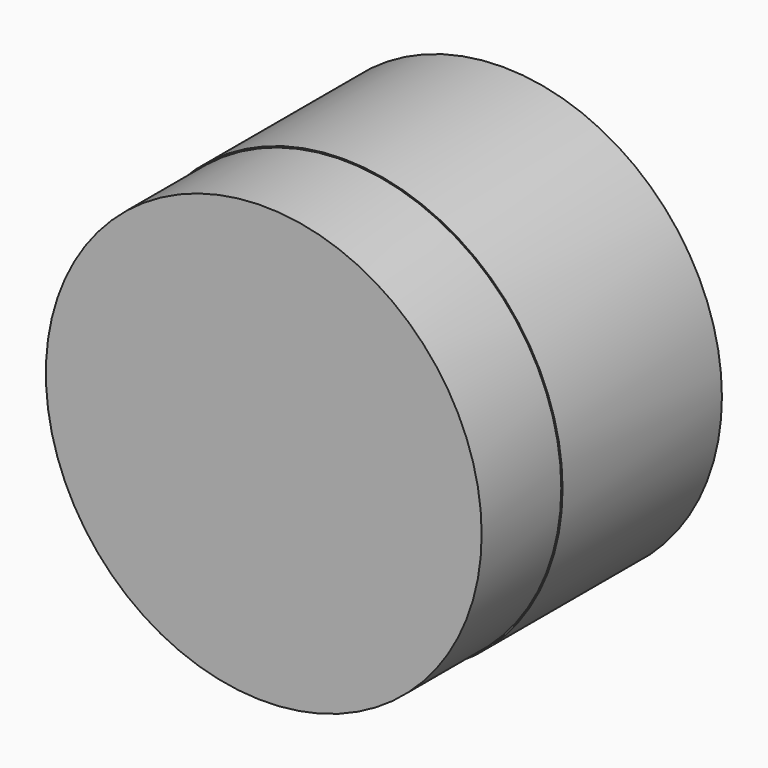
from build123d import *

# Parameters (mm, degrees)
F1_START = 20
F0_R     = 44
F0_R_2   = 30
F1_DEPTH = 40
F3_START = 60.01
F2_R     = 43.7564133354
F3_DEPTH = 19.99


with BuildPart() as f1:
    # F0 (on Front) → F1 (new body)
    with BuildSketch(Plane.XZ.offset(F1_START)):
        Circle(F0_R)
        Circle(F0_R_2, mode=Mode.SUBTRACT)
    extrude(amount=F1_DEPTH)


with BuildPart() as f3:
    # F2 (on Front) → F3 (new body)
    with BuildSketch(Plane.XZ.offset(F3_START)):
        Circle(F2_R)
    extrude(amount=F3_DEPTH)


solid = Compound([f1.part, f3.part])
